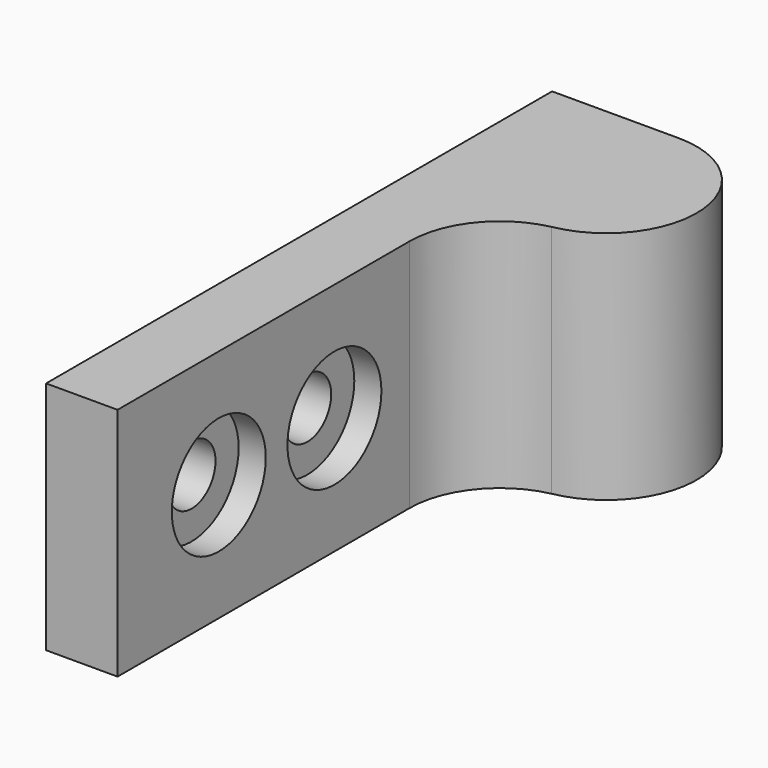
from build123d import *

# Parameters (mm, degrees)
F1_DEPTH       = 13
F2_T1_DEPTH    = 13
F4_D           = 3.3
F4_CBORE_D     = 6.5
F4_CBORE_DEPTH = 1.5


# Not quite as in the source:
# - a fillet or chamfer that OpenCascade refuses, or shapes differently, is made with other operations: its cross-section is extruded or revolved along the edge and cut away or added


with BuildPart() as f1:
    # F0 (on Top) → F1 (new body)
    with BuildSketch(Plane.XY):
        with BuildLine():
            Line((6.184642151, 5.8486273885), (-0.815357849, 5.8486273885))
            Line((-0.815357849, 5.8486273885), (-0.815357849, -29.1513726115))
            Line((-0.815357849, -29.1513726115), (3.1407309243, -29.1513726115))
            Line((3.1407309243, -29.1513726115), (3.1407309243, -4.0674617201))
            Line((3.1407309243, -4.0674617201), (7.0968196975, -4.0674617201))
            ThreePointArc((7.0968196975, -4.0674617201), (11.1636202361, 1.3066418299), (6.184642151, 5.8486273885))
        make_face()
    extrude(amount=F1_DEPTH)

    # F2: fillet of radius 5 on 1 edges, made by hand

    # F2_s2 → F2_t1 (join)
    with BuildSketch(Plane.XY):
        with BuildLine():
            ThreePointArc((7.0968196975, -4.0674617201), (4.2536011262, -5.8124001647), (3.1407309243, -8.9572724885))
            Line((3.1407309243, -8.9572724885), (3.1407309243, -4.0674617201))
            Line((3.1407309243, -4.0674617201), (7.0968196975, -4.0674617201))
        make_face()
    extrude(amount=F2_T1_DEPTH)

    # F4 (through all)
    with Locations(Plane.YZ.offset(3.1407309243)):
        with Locations((-22.1513726115, 6.5), (-14.1513726115, 6.5)):
            CounterBoreHole(F4_D / 2, F4_CBORE_D / 2, F4_CBORE_DEPTH)


solid = f1.part
